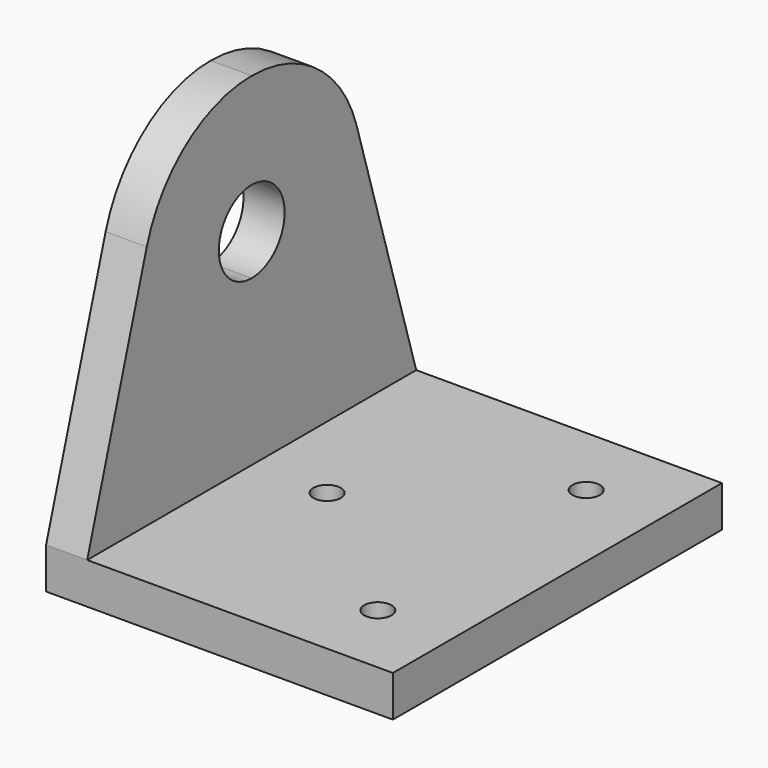
from build123d import *

# Parameters (mm, degrees)
F0_W     = 25.3
F0_H     = 30
F1_DEPTH = 3
F2_W     = 3
F2_H     = 30
F3_DEPTH = 25
F5_DEPTH = 3
F6_R     = 1
F7_DEPTH = 3


# Not quite as in the source:
# - a feature names something its author has since deleted; it is built from what else it names


with BuildPart() as f1:
    # F0 (on Top) → F1 (new body)
    with BuildSketch(Plane.XY):
        Rectangle(F0_W, F0_H)
    extrude(amount=-F1_DEPTH)

    # F2 (on face) → F3 (join)
    with BuildSketch(Plane.XY):
        with Locations((-11.15, 0)):
            Rectangle(F2_W, F2_H)
    extrude(amount=F3_DEPTH)

    # F4 (on face) → F5 (cut)
    with BuildSketch(Plane(origin=(-12.65, 0, 0), x_dir=(0, -1, 0), z_dir=(-1, 0, 0))):
        with BuildLine():
            ThreePointArc((3, 15), (-2.1213203436, 17.1213203436), (0, 12))
            ThreePointArc((0, 12), (2.1213203436, 12.8786796564), (3, 15))
        make_face()
        with BuildLine():
            Line((-15, 25), (-15, 0))
            Line((-15, 0), (-9.569428978, 17.9027623113))
            ThreePointArc((-9.569428978, 17.9027623113), (-5.9570284911, 23.032049026), (0, 25))
            Line((0, 25), (-15, 25))
        make_face()
        with BuildLine():
            Line((9.569428978, 17.9027623113), (15, 0))
            Line((15, 0), (15, 25))
            Line((15, 25), (0, 25))
            ThreePointArc((0, 25), (5.9570284911, 23.032049026), (9.569428978, 17.9027623113))
        make_face()
    extrude(amount=-F5_DEPTH, mode=Mode.SUBTRACT)

    # F6 (on face) → F7 (cut)
    with BuildSketch(Plane.XY):
        with Locations((7.15, -9.5)):
            Circle(F6_R)
        with Locations((-4.15, 0)):
            Circle(F6_R)
        with Locations((7.15, 9.5)):
            Circle(F6_R)
    extrude(amount=-F7_DEPTH, mode=Mode.SUBTRACT)


solid = f1.part
